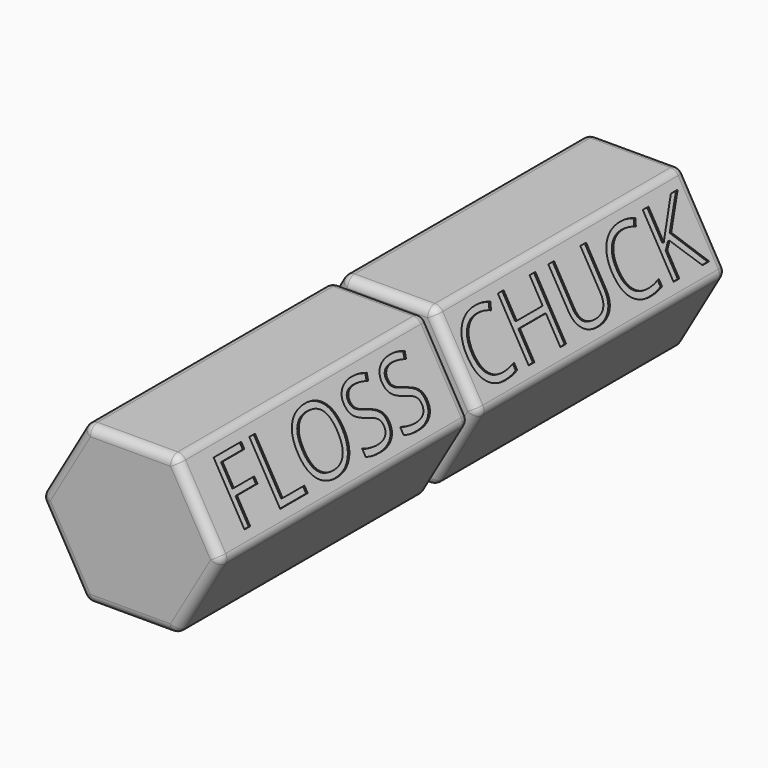
from build123d import *

# Parameters (mm, degrees)
F1_DEPTH     = 44.45
F2_R         = 14.1735226281
F2_R_2       = 7.8235222027
F3_DEPTH     = 0.635
F4_SIZE      = 0.63499
F5_R         = 1.27
F6_R         = 1.27
F7_TEXT_SIZE = 12.1174311927
F8_DEPTH     = 0.25


# Not quite as in the source:
# - a fillet or chamfer is up to 0.001 mm smaller than in the source, because OpenCascade refuses the exact size
# - Text() gives the source's letters only with a copy of the font that has no kerning and outlines rounded to 1/6400 em; it was checked with that copy


with BuildPart() as f1:
    # F0 (on Front) → F1 (new body, symmetric)
    with BuildSketch(Plane.XZ):
        with BuildLine():
            Line((6.7166174209, -10.3635226281), (12.3333825791, -0.635))
            ThreePointArc((12.3333825791, -0.635), (12.5035303163, 0), (12.3333825791, 0.635))
            Line((12.3333825791, 0.635), (6.7166174209, 10.3635226281))
            ThreePointArc((6.7166174209, 10.3635226281), (6.2517651581, 10.8283748909), (5.6167651581, 10.9985226281))
            Line((5.6167651581, 10.9985226281), (-5.6167651581, 10.9985226281))
            ThreePointArc((-5.6167651581, 10.9985226281), (-6.2517651581, 10.8283748909), (-6.7166174209, 10.3635226281))
            Line((-6.7166174209, 10.3635226281), (-12.3333825791, 0.635))
            ThreePointArc((-12.3333825791, 0.635), (-12.5035303163, 0), (-12.3333825791, -0.635))
            Line((-12.3333825791, -0.635), (-6.7166174209, -10.3635226281))
            ThreePointArc((-6.7166174209, -10.3635226281), (-6.2517651581, -10.8283748909), (-5.6167651581, -10.9985226281))
            Line((-5.6167651581, -10.9985226281), (5.6167651581, -10.9985226281))
            ThreePointArc((5.6167651581, -10.9985226281), (6.2517651581, -10.8283748909), (6.7166174209, -10.3635226281))
        make_face()
    extrude(amount=F1_DEPTH, both=True)

    # F2 (on Front) → F3 (cut, symmetric)
    with BuildSketch(Plane.XZ):
        Circle(F2_R)
        Circle(F2_R_2, mode=Mode.SUBTRACT)
    extrude(amount=F3_DEPTH, both=True, mode=Mode.SUBTRACT)

    # F4 (size 0.635 in the source; OpenCascade refuses exactly that, so slightly less here)
    f4_edges = [f1.edges().sort_by_distance(p)[0] for p in [
        (-7.823522, -0.635, 0),
        (7.823522, 0, 0),
        (-7.823522, 0.635, 0),
    ]]
    chamfer(f4_edges, length=F4_SIZE)

    # F5
    f5_edges = [f1.edges().sort_by_distance(p)[0] for p in [
        (0, 0.635, -10.998523),
        (0, -0.635, -10.998523),
    ]]
    fillet(f5_edges, radius=F5_R)

    # F6
    f6_edges = [f1.edges().sort_by_distance(p)[0] for p in [
        (0, -44.45, -10.998523),
        (0, 44.45, -10.998523),
    ]]
    fillet(f6_edges, radius=F6_R)

    # F7 (on face) → F8 (cut)
    with BuildSketch(Plane(origin=(9.525, 0, 5.499261314), x_dir=(0, 1, 0), z_dir=(0.8660254038, 0, 0.5))):
        with Locations((-40.2860166284, -4.3622752294)):
            Text('FLOSS', F7_TEXT_SIZE, font='Open Sans', text_align=(TextAlign.LEFT, TextAlign.BOTTOM))
        with Locations((1.905, -4.3622752294)):
            Text('CHUCK', F7_TEXT_SIZE, font='Open Sans', text_align=(TextAlign.LEFT, TextAlign.BOTTOM))
    extrude(amount=-F8_DEPTH, mode=Mode.SUBTRACT)


solid = f1.part
